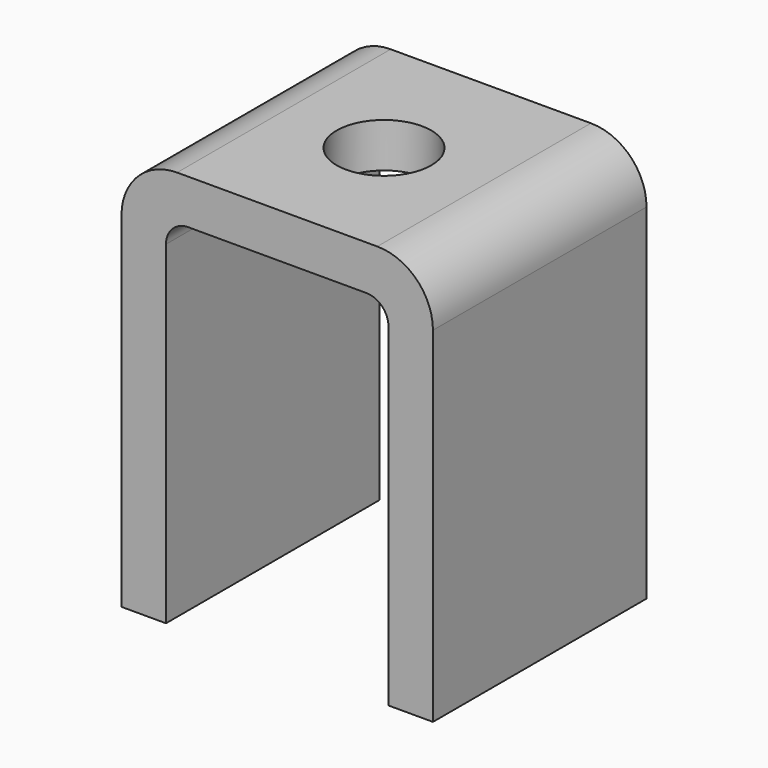
from build123d import *

# Parameters (mm, degrees)
F1_DEPTH = 38.1
F2_R     = 6.35
F3_R     = 15.875
F4_R     = 13.49375
F5_DEPTH = 57.151


with BuildPart() as f1:
    # F0 (on Front) → F1 (new body, symmetric)
    with BuildSketch(Plane.XZ):
        Polygon((31.75, -57.15), (44.45, -57.15), (44.45, 57.15), (-44.45, 57.15), (-44.45, -57.15), (-31.75, -57.15), (-31.75, 44.45), (31.75, 44.45), align=None)
    extrude(amount=F1_DEPTH, both=True)

    # F2
    f2_edges = [f1.edges().sort_by_distance(p)[0] for p in [
        (-31.75, 0, 44.45),
        (31.75, 0, 44.45),
    ]]
    fillet(f2_edges, radius=F2_R)

    # F3
    f3_edges = [f1.edges().sort_by_distance(p)[0] for p in [
        (-44.45, 0, 57.15),
        (44.45, 0, 57.15),
    ]]
    fillet(f3_edges, radius=F3_R)

    # F4 (on Top) → F5 (cut, through all)
    with BuildSketch(Plane.XY):
        Circle(F4_R)
    extrude(amount=F5_DEPTH, mode=Mode.SUBTRACT)


solid = f1.part
